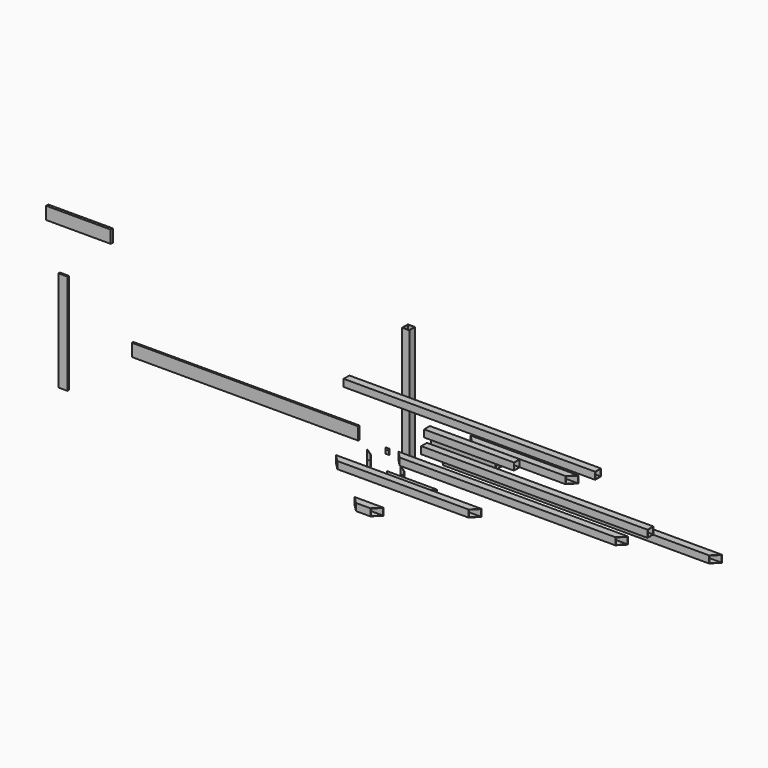
from build123d import *

# Parameters (mm, degrees)
F0_W         = 50.8
F0_H         = 50.8
F0_W_2       = 46.5836
F0_H_2       = 46.5836
F1_DEPTH     = 838.2
F2_W         = 50.8
F2_H         = 50.8
F2_W_2       = 46.5836
F2_H_2       = 46.5836
F3_DEPTH     = 1600.2
F4_W         = 50.8
F4_H         = 50.8
F4_W_2       = 46.5836
F4_H_2       = 46.5836
F5_DEPTH     = 457.2
F6_W         = 50.8
F6_H         = 50.8
F6_W_2       = 46.5836
F6_H_2       = 46.5836
F7_DEPTH     = 1981.2
F9_DEPTH     = 50.8
F10_W        = 50.8
F10_H        = 50.8
F10_W_2      = 46.5836
F10_H_2      = 46.5836
F11_DEPTH    = 762
F13_DEPTH    = 50.8
F14_R        = 2.38125
F15_DEPTH    = 3.175
F16_W        = 25.4
F16_H        = 25.4
F16_R        = 2.38125
F17_DEPTH    = 3.175
F18_W        = 1600.2
F18_H        = 88.9
F19_DEPTH    = 12.7
F20_W        = 63.5
F20_H        = 711.2
F21_DEPTH    = 12.7
F22_W        = 50.8
F22_H        = 50.8
F22_W_2      = 46.5836
F22_H_2      = 46.5836
F23_DEPTH    = 355.6
F24_T1_DEPTH = 312.0829915773
F25_W        = 50.8
F25_H        = 50.8
F25_W_2      = 46.5836
F25_H_2      = 46.5836
F26_DEPTH    = 1625.6
F27_T1_DEPTH = 312.0829915773
F28_W        = 50.8
F28_H        = 50.8
F28_W_2      = 46.5836
F28_H_2      = 46.5836
F29_DEPTH    = 203.2
F30_T1_DEPTH = 312.0829915773
F31_R        = 2.38125
F32_DEPTH    = 3.175
F33_W        = 25.4
F33_H        = 38.1
F33_R        = 2.38125
F34_DEPTH    = 3.175
F35_W        = 457.2
F35_H        = 88.9
F36_DEPTH    = 19.05
F37_W        = 50.8
F37_H        = 50.8
F37_W_2      = 46.5836
F37_H_2      = 46.5836
F38_DEPTH    = 1028.7
F39_T1_DEPTH = 312.0829915773
F40_W        = 50.8
F40_H        = 50.8
F40_W_2      = 46.5836
F40_H_2      = 46.5836
F41_DEPTH    = 635
F42_W        = 50.8
F42_H        = 50.8
F42_W_2      = 46.5836
F42_H_2      = 46.5836
F43_DEPTH    = 1778


# Not quite as in the source:
# - a fillet or chamfer that OpenCascade refuses, or shapes differently, is made with other operations: its cross-section is extruded or revolved along the edge and cut away or added


with BuildPart() as f1:
    # F0 (on Top) → F1 (new body)
    with BuildSketch(Plane.XY):
        with Locations((-23.9895193481, -62.8970144058)):
            Rectangle(F0_W, F0_H)
        with Locations((-23.9895193481, -62.8970144058)):
            Rectangle(F0_W_2, F0_H_2, mode=Mode.SUBTRACT)
    extrude(amount=F1_DEPTH)


with BuildPart() as f3:
    # F2 (on Right) → F3 (new body)
    with BuildSketch(Plane.YZ):
        with Locations((43.8489612991, 48.4097724301)):
            Rectangle(F2_W, F2_H)
        with Locations((43.8489612991, 48.4097724301)):
            Rectangle(F2_W_2, F2_H_2, mode=Mode.SUBTRACT)
    extrude(amount=F3_DEPTH)


with BuildPart() as f5:
    # F4 (on Right) → F5 (new body)
    with BuildSketch(Plane.YZ):
        with Locations((129.718255794, 63.5042605758)):
            Rectangle(F4_W, F4_H)
        with Locations((129.718255794, 63.5042605758)):
            Rectangle(F4_W_2, F4_H_2, mode=Mode.SUBTRACT)
    extrude(amount=F5_DEPTH)


with BuildPart() as f7:
    # F6 (on Right) → F7 (new body)
    with BuildSketch(Plane.YZ):
        with Locations((174.2987973452, -56.7749696016)):
            Rectangle(F6_W, F6_H)
        with Locations((174.2987973452, -56.7749696016)):
            Rectangle(F6_W_2, F6_H_2, mode=Mode.SUBTRACT)
    extrude(amount=F7_DEPTH)

    # F8 (on face) → F9 (cut, through all)
    with BuildSketch(Plane.XY.offset(-31.3749696016)):
        Polygon((1981.2, 148.8987973452), (1981.2, 199.6987973452), (1930.4, 148.8987973452), align=None)
        Polygon((50.8, 148.8987973452), (0, 199.6987973452), (0, 148.8987973452), align=None)
    extrude(amount=-F9_DEPTH, mode=Mode.SUBTRACT)


with BuildPart() as f11:
    # F10 (on Right) → F11 (new body)
    with BuildSketch(Plane.YZ):
        with Locations((429.6248448849, -63.3640619159)):
            Rectangle(F10_W, F10_H)
        with Locations((429.6248448849, -63.3640619159)):
            Rectangle(F10_W_2, F10_H_2, mode=Mode.SUBTRACT)
    extrude(amount=F11_DEPTH)

    # F12 (on face) → F13 (cut, through all)
    with BuildSketch(Plane.XY.offset(-37.9640619159)):
        Polygon((50.8, 404.2248448849), (0, 455.0248448849), (0, 404.2248448849), align=None)
        Polygon((762, 404.2248448849), (762, 455.0248448849), (711.2, 404.2248448849), align=None)
    extrude(amount=-F13_DEPTH, mode=Mode.SUBTRACT)


with BuildPart() as f15:
    # F14 (on Front) → F15 (new body)
    with BuildSketch(Plane.XZ):
        Polygon((-103.7242509466, -109.7514086127), (-129.1242509466, -84.3514086127), (-129.1242509466, -185.9514086127), (-103.7242509466, -160.5514086127), align=None)
        with Locations((-116.4242509466, -135.1514086127)):
            Circle(F14_R, mode=Mode.SUBTRACT)
    extrude(amount=F15_DEPTH)


with BuildPart() as f17:
    # F16 (on Front) → F17 (new body)
    with BuildSketch(Plane.XZ):
        with Locations((9.3765241186, -168.3152318001)):
            Rectangle(F16_W, F16_H)
        with Locations((9.3765241186, -168.3152318001)):
            Circle(F16_R, mode=Mode.SUBTRACT)
    extrude(amount=F17_DEPTH)


with BuildPart() as f19:
    # F18 (on Front) → F19 (new body)
    with BuildSketch(Plane.XZ):
        with Locations((-1220.8474673271, 28.1916467965)):
            Rectangle(F18_W, F18_H)
    extrude(amount=F19_DEPTH)


with BuildPart() as f21:
    # F20 (on Front) → F21 (new body)
    with BuildSketch(Plane.XZ):
        with Locations((-2507.8683080673, -19.528626181)):
            Rectangle(F20_W, F20_H)
    extrude(amount=F21_DEPTH)


with BuildPart() as f23:
    # F22 (on Right) → F23 (new body)
    with BuildSketch(Plane.YZ):
        with Locations((-311.0560774803, 17.0110743493)):
            Rectangle(F22_W, F22_H)
        with Locations((-311.0560774803, 17.0110743493)):
            Rectangle(F22_W_2, F22_H_2, mode=Mode.SUBTRACT)
    extrude(amount=F23_DEPTH)

    # F24: chamfer of 50.8 on 2 edges, made by hand

    # F24_s2 → F24_t1 (cut)
    with BuildSketch(Plane.XY.offset(-139.0304214394)):
        Polygon((304.8, -336.4560774803), (355.6, -285.6560774803), (355.6, -336.4560774803), align=None)
        Polygon((50.8, -336.4560774803), (0, -285.6560774803), (0, -336.4560774803), align=None)
    extrude(amount=F24_T1_DEPTH, mode=Mode.SUBTRACT)


with BuildPart() as f26:
    # F25 (on Right) → F26 (new body)
    with BuildSketch(Plane.YZ):
        with Locations((-209.4067037106, 96.6901108623)):
            Rectangle(F25_W, F25_H)
        with Locations((-209.4067037106, 96.6901108623)):
            Rectangle(F25_W_2, F25_H_2, mode=Mode.SUBTRACT)
    extrude(amount=F26_DEPTH)

    # F27: chamfer of 50.8 on 2 edges, made by hand

    # F27_s2 → F27_t1 (cut)
    with BuildSketch(Plane.XY.offset(-59.3513849264)):
        Polygon((50.8, -234.8067037106), (0, -184.0067037106), (0, -234.8067037106), align=None)
        Polygon((1574.8, -234.8067037106), (1625.6, -184.0067037106), (1625.6, -234.8067037106), align=None)
    extrude(amount=F27_T1_DEPTH, mode=Mode.SUBTRACT)


with BuildPart() as f29:
    # F28 (on Right) → F29 (new body)
    with BuildSketch(Plane.YZ):
        with Locations((-595.3577756882, -29.1252676398)):
            Rectangle(F28_W, F28_H)
        with Locations((-595.3577756882, -29.1252676398)):
            Rectangle(F28_W_2, F28_H_2, mode=Mode.SUBTRACT)
    extrude(amount=F29_DEPTH)

    # F30: chamfer of 50.8 on 2 edges, made by hand

    # F30_s2 → F30_t1 (cut)
    with BuildSketch(Plane.XY.offset(-185.1667634284)):
        Polygon((152.4, -620.7577756882), (203.2, -569.9577756882), (203.2, -620.7577756882), align=None)
        Polygon((50.8, -620.7577756882), (0, -569.9577756882), (0, -620.7577756882), align=None)
    extrude(amount=F30_T1_DEPTH, mode=Mode.SUBTRACT)


with BuildPart() as f32:
    # F31 (on Front) → F32 (new body)
    with BuildSketch(Plane.XZ):
        Polygon((-339.7773418903, -82.8328536272), (-365.1773418903, -57.4328536272), (-365.1773418903, -184.4328536272), (-339.7773418903, -159.0328536272), align=None)
        with Locations((-352.4773418903, -120.9328536272)):
            Circle(F31_R, mode=Mode.SUBTRACT)
    extrude(amount=F32_DEPTH)


with BuildPart() as f34:
    # F33 (on Front) → F34 (new body)
    with BuildSketch(Plane.XZ):
        with Locations((-222.7736711502, -22.2336029798)):
            Rectangle(F33_W, F33_H)
        with Locations((-222.7736711502, -15.8836029798)):
            Circle(F33_R, mode=Mode.SUBTRACT)
    extrude(amount=F34_DEPTH)


with BuildPart() as f36:
    # F35 (on Front) → F36 (new body)
    with BuildSketch(Plane.XZ):
        with Locations((-2393.2858118057, 687.9762411118)):
            Rectangle(F35_W, F35_H)
    extrude(amount=F36_DEPTH)


with BuildPart() as f38:
    # F37 (on Right) → F38 (new body)
    with BuildSketch(Plane.YZ):
        with Locations((-760.5085968971, 299.0830242634)):
            Rectangle(F37_W, F37_H)
        with Locations((-760.5085968971, 299.0830242634)):
            Rectangle(F37_W_2, F37_H_2, mode=Mode.SUBTRACT)
    extrude(amount=F38_DEPTH)

    # F39: chamfer of 50.8 on 2 edges, made by hand

    # F39_s2 → F39_t1 (cut)
    with BuildSketch(Plane.XY.offset(143.0415284747)):
        Polygon((977.9, -785.9085968971), (1028.7, -735.1085968971), (1028.7, -785.9085968971), align=None)
        Polygon((50.8, -785.9085968971), (0, -735.1085968971), (0, -785.9085968971), align=None)
    extrude(amount=F39_T1_DEPTH, mode=Mode.SUBTRACT)


with BuildPart() as f41:
    # F40 (on Right) → F41 (new body)
    with BuildSketch(Plane.YZ):
        with Locations((69.8824599385, 142.1617567539)):
            Rectangle(F40_W, F40_H)
        with Locations((69.8824599385, 142.1617567539)):
            Rectangle(F40_W_2, F40_H_2, mode=Mode.SUBTRACT)
    extrude(amount=F41_DEPTH)


with BuildPart() as f43:
    # F42 (on Right) → F43 (new body)
    with BuildSketch(Plane.YZ):
        with Locations((-641.3798928261, 745.8674311638)):
            Rectangle(F42_W, F42_H)
        with Locations((-641.3798928261, 745.8674311638)):
            Rectangle(F42_W_2, F42_H_2, mode=Mode.SUBTRACT)
    extrude(amount=F43_DEPTH)


solid = Compound([f1.part, f3.part, f5.part, f7.part, f11.part, f15.part, f17.part, f19.part, f21.part, f23.part, f26.part, f29.part, f32.part, f34.part, f36.part, f38.part, f41.part, f43.part])
